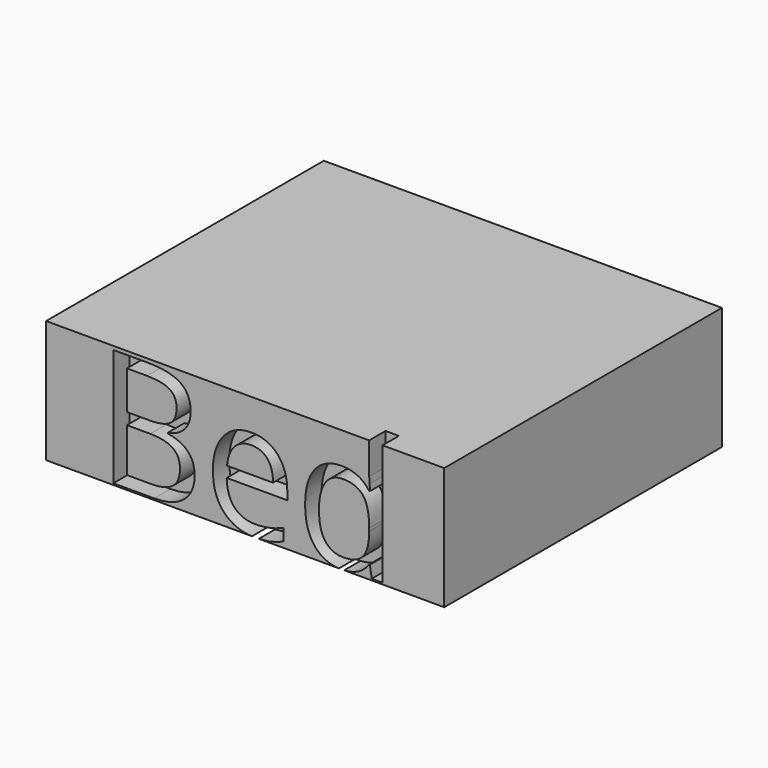
from build123d import *

# Parameters (mm, degrees)
F0_W         = 495.3
F0_H         = 152.4
F1_DEPTH     = 431.8
F2_TEXT_SIZE = 204.5223427332
F3_DEPTH     = 25.4


# Not quite as in the source:
# - Text() gives the source's letters only with a copy of the font that has no kerning and outlines rounded to 1/6400 em; it was checked with that copy


with BuildPart() as f1:
    # F0 (on Front) → F1 (new body)
    with BuildSketch(Plane.XZ):
        Rectangle(F0_W, F0_H)
    extrude(amount=F1_DEPTH)

    # F2 (on face) → F3 (cut)
    with BuildSketch(Plane.XZ.offset(431.8)):
        with Locations((-184.15, -74.2725988267)):
            Text('Bed', F2_TEXT_SIZE, font='Open Sans', text_align=(TextAlign.LEFT, TextAlign.BOTTOM))
    extrude(amount=-F3_DEPTH, mode=Mode.SUBTRACT)


solid = f1.part
